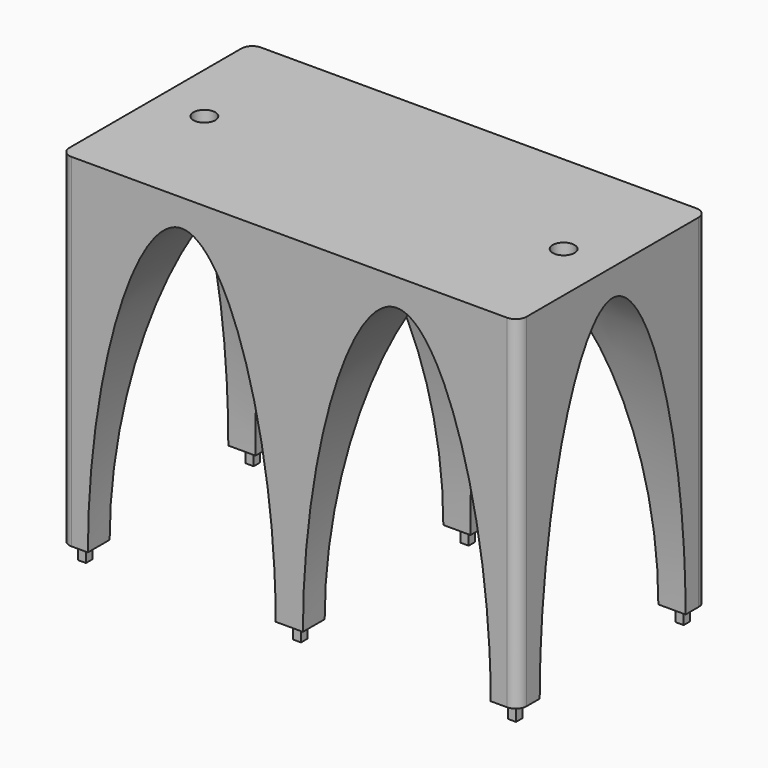
from build123d import *

# Parameters (mm, degrees)
F0_W      = 43.5
F0_H      = 3
F1_DEPTH  = 84
F3_DEPTH  = 84
F5_DEPTH  = 43.5
F6_R      = 2
F7_R      = 2
F8_DEPTH  = 4
F9_W      = 1.5
F9_H      = 1.5
F10_DEPTH = 3


# Not quite as in the source:
# - a feature names something its author has since deleted; it is built from what else it names


with BuildPart() as f1:
    # F0 (on Right) → F1 (new body)
    with BuildSketch(Plane.YZ):
        with Locations((21.75, 64.5)):
            Rectangle(F0_W, F0_H)
        Polygon((0, 63), (0, 3), (21, 3), (43.5, 3), (43.5, 63), align=None)
    extrude(amount=-F1_DEPTH)

    # F2 (on Right) → F3 (cut, through all)
    with BuildSketch(Plane.YZ):
        with BuildLine():
            add(Edge.make_bspline(
                [(4.9999998882, 3), (4.9999998882, 32.0000000559), (21.75, 90.0000001676), (38.5000001118, 32.0000000559), (38.5000001118, 3)],
                knots=[0, 0, 0, 0, 0.5, 1, 1, 1, 1], degree=3))
            Line((4.9999998882, 3), (38.5000001118, 3))
        make_face()
    extrude(amount=-F3_DEPTH, mode=Mode.SUBTRACT)

    # F4 (on Front) → F5 (cut, through all)
    with BuildSketch(Plane.XZ):
        with BuildLine():
            add(Edge.make_bspline(
                [(-79.0000001118, 3), (-79.0000001118, 32.0000000559), (-61.7500000559, 90.0000001676), (-44.5, 32.0000000559), (-44.5, 3)],
                knots=[0, 0, 0, 0, 0.5, 1, 1, 1, 1], degree=3))
            Line((-79.0000001118, 3), (-44.5, 3))
        make_face()
        with BuildLine():
            add(Edge.make_bspline(
                [(-39.5, 3), (-39.5, 32.0000000559), (-22.2499999441, 90.0000001676), (-4.9999998882, 32.0000000559), (-4.9999998882, 3)],
                knots=[0, 0, 0, 0, 0.5, 1, 1, 1, 1], degree=3))
            Line((-39.5, 3), (-4.9999998882, 3))
        make_face()
    extrude(amount=-F5_DEPTH, mode=Mode.SUBTRACT)

    # F6
    f6_edges = [f1.edges().sort_by_distance(p)[0] for p in [
        (0, 0, 34.5),
        (-84, 0, 34.5),
        (0, 43.5, 34.5),
        (-84, 43.5, 34.5),
    ]]
    fillet(f6_edges, radius=F6_R)

    # F7 (on face) → F8 (cut)
    with BuildSketch(Plane.XY.offset(66)):
        with Locations((-75, 21.75)):
            Circle(F7_R)
        with Locations((-9, 21.75)):
            Circle(F7_R)
    extrude(amount=-F8_DEPTH, mode=Mode.SUBTRACT)

    # F9 (on face) → F10 (join)
    with BuildSketch(Plane(origin=(0, 0, 3), x_dir=(1, 0, 0), z_dir=(0, 0, -1))):
        with Locations((-42, -2.4999999446)):
            Rectangle(F9_W, F9_H)
        with Locations((-2.4999999441, -2.4999999444)):
            Rectangle(F9_W, F9_H)
        with Locations((-2.4999999443, -41.0000000559)):
            Rectangle(F9_W, F9_H)
        with Locations((-42, -41.0000000564)):
            Rectangle(F9_W, F9_H)
        with Locations((-81.5000000559, -41.0000000561)):
            Rectangle(F9_W, F9_H)
        with Locations((-81.5000000562, -2.4999999441)):
            Rectangle(F9_W, F9_H)
    extrude(amount=F10_DEPTH)


solid = f1.part
